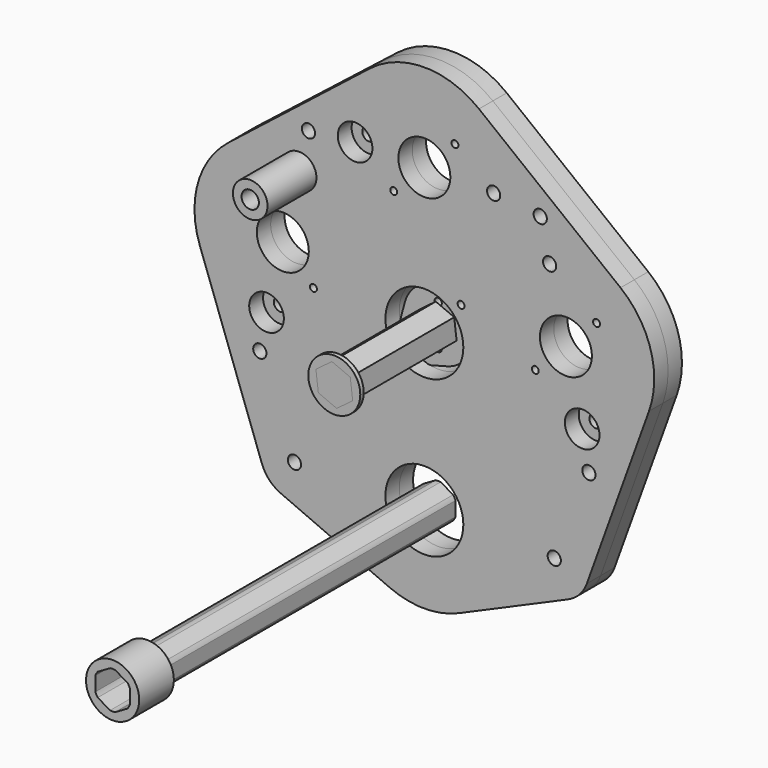
from build123d import *

# Parameters (mm, degrees)
F0_R      = 2.4257
F0_R_2    = 1.27
F0_R_3    = 14.2875
F0_R_4    = 9.525
F1_DEPTH  = 6.35
F2_R      = 6.35
F2_R_2    = 3.175
F3_DEPTH  = 28.7528
F5_DEPTH  = 47.625
F6_R      = 2.5527
F7_DEPTH  = 133.35
F8_R      = 2.4257
F8_R_2    = 6.35
F8_R_3    = 1.27
F8_R_4    = 14.2875
F8_R_5    = 9.525
F9_DEPTH  = 6.35
F10_R     = 9.7536
F11_DEPTH = 15.875
F12_R     = 9.525
F13_DEPTH = 1.5875
F14_R     = 1.3208
F14_R_2   = 1.27
F14_R_3   = 4.7625
F15_DEPTH = 3.175
F16_R     = 3.175
F16_R_2   = 1.27
F17_DEPTH = 6.35


with BuildPart() as f1:
    # F0 (on Front) → F1 (new body)
    with BuildSketch(Plane.XZ):
        with BuildLine():
            ThreePointArc((20.0287821123, 78.8394956856), (0, 85.7758), (-20.0287821123, 78.8394956856))
            Line((-20.0287821123, 78.8394956856), (-71.9241615496, 37.9964890253))
            ThreePointArc((-71.9241615496, 37.9964890253), (-83.0312055128, 21.4555741857), (-82.3532815297, 1.5430477664))
            Line((-82.3532815297, 1.5430477664), (-59.5692753303, -61.5163864993))
            ThreePointArc((-59.5692753303, -61.5163864993), (-56.8914611396, -65.8854242261), (-52.705, -68.8405422652))
            Line((-52.705, -68.8405422652), (-12.7, -86.300155663))
            ThreePointArc((-12.7, -86.300155663), (0, -88.9508), (12.7, -86.300155663))
            Line((12.7, -86.300155663), (52.705, -68.8405422652))
            ThreePointArc((52.705, -68.8405422652), (56.8914611396, -65.8854242261), (59.5692753303, -61.5163864993))
            Line((59.5692753303, -61.5163864993), (82.3532815297, 1.5430477664))
            ThreePointArc((82.3532815297, 1.5430477664), (83.0312055128, 21.4555741857), (71.9241615496, 37.9964890253))
            Line((71.9241615496, 37.9964890253), (20.0287821123, 78.8394956856))
        make_face()
        with Locations((-47.625, -57.2008)):
            Circle(F0_R, mode=Mode.SUBTRACT)
        with Locations((-60.325, -25.4508)):
            Circle(F0_R, mode=Mode.SUBTRACT)
        with Locations((-57.8648339281, -12.1407791805)):
            Circle(F0_R, mode=Mode.SUBTRACT)
        with Locations((-13.4703841816, -13.4703841816)):
            Circle(F0_R_2, mode=Mode.SUBTRACT)
        with Locations((0, -57.2008)):
            Circle(F0_R_3, mode=Mode.SUBTRACT)
        with Locations((47.625, -57.2008)):
            Circle(F0_R, mode=Mode.SUBTRACT)
        with Locations((60.325, -25.4508)):
            Circle(F0_R, mode=Mode.SUBTRACT)
        with Locations((57.8648339281, -12.1407791805)):
            Circle(F0_R, mode=Mode.SUBTRACT)
        with Locations((-51.8953794373, 12.5477933397)):
            Circle(F0_R_4, mode=Mode.SUBTRACT)
        with Locations((-63.1206995887, 23.773113491)):
            Circle(F0_R_2, mode=Mode.SUBTRACT)
        with Locations((-45.9259249465, 37.2363658598)):
            Circle(F0_R, mode=Mode.SUBTRACT)
        with Locations((-40.670059286, 1.3224731883)):
            Circle(F0_R_2, mode=Mode.SUBTRACT)
        with Locations((-42.4934886143, 51.4322950589)):
            Circle(F0_R, mode=Mode.SUBTRACT)
        with Locations((-25.4, 53.3908)):
            Circle(F0_R, mode=Mode.SUBTRACT)
        with Locations((-11.2253201513, 42.1654798487)):
            Circle(F0_R_2, mode=Mode.SUBTRACT)
        Circle(F0_R_3, mode=Mode.SUBTRACT)
        with Locations((13.4703841816, 13.4703841816)):
            Circle(F0_R_2, mode=Mode.SUBTRACT)
        with Locations((40.670059286, 1.3224731883)):
            Circle(F0_R_2, mode=Mode.SUBTRACT)
        with Locations((51.8953794373, 12.5477933397)):
            Circle(F0_R_4, mode=Mode.SUBTRACT)
        with Locations((63.1206995887, 23.773113491)):
            Circle(F0_R_2, mode=Mode.SUBTRACT)
        with Locations((45.9259249465, 37.2363658598)):
            Circle(F0_R, mode=Mode.SUBTRACT)
        with Locations((0, 53.3908)):
            Circle(F0_R_4, mode=Mode.SUBTRACT)
        with Locations((25.4, 53.3908)):
            Circle(F0_R, mode=Mode.SUBTRACT)
        with Locations((11.2253201513, 64.6161201513)):
            Circle(F0_R_2, mode=Mode.SUBTRACT)
        with Locations((42.4934886143, 51.4322950589)):
            Circle(F0_R, mode=Mode.SUBTRACT)
    extrude(amount=F1_DEPTH)


with BuildPart() as f3:
    # F2 (on face) → F3 (new body)
    with BuildSketch(Plane.XZ.offset(6.35)):
        with Locations((-45.9259249465, 37.2363658598)):
            Circle(F2_R)
        with Locations((-45.9259249465, 37.2363658598)):
            Circle(F2_R_2, mode=Mode.SUBTRACT)
    extrude(amount=F3_DEPTH)


with BuildPart() as f5:
    # F4 (on face) → F5 (new body)
    with BuildSketch(Plane.XZ.offset(6.35)):
        Polygon((0.8878003498, -7.2784025632), (6.7471816936, -2.8703436252), (5.8593813438, 4.408058938), (-0.8878003498, 7.2784025632), (-6.7471816936, 2.8703436252), (-5.8593813438, -4.408058938), align=None)
    extrude(amount=F5_DEPTH)


with BuildPart() as f7:
    # F6 (on face) → F7 (new body)
    with BuildSketch(Plane.XZ.offset(6.35)):
        with BuildLine():
            Line((0.8930394942, -64.0175518263), (5.4569605058, -61.3825708017))
            ThreePointArc((5.4569605058, -61.3825708017), (5.953924651, -60.6383), (6.35, -59.8357810246))
            Line((6.35, -59.8357810246), (6.35, -54.5658189754))
            ThreePointArc((6.35, -54.5658189754), (5.953924651, -53.7633), (5.4569605058, -53.0190291983))
            Line((5.4569605058, -53.0190291983), (0.8930394942, -50.3840481737))
            ThreePointArc((0.8930394942, -50.3840481737), (0, -50.3258), (-0.8930394942, -50.3840481737))
            Line((-0.8930394942, -50.3840481737), (-5.4569605058, -53.0190291983))
            ThreePointArc((-5.4569605058, -53.0190291983), (-5.953924651, -53.7633), (-6.35, -54.5658189754))
            Line((-6.35, -54.5658189754), (-6.35, -59.8357810246))
            ThreePointArc((-6.35, -59.8357810246), (-5.953924651, -60.6383), (-5.4569605058, -61.3825708017))
            Line((-5.4569605058, -61.3825708017), (-0.8930394942, -64.0175518263))
            ThreePointArc((-0.8930394942, -64.0175518263), (0, -64.0758), (0.8930394942, -64.0175518263))
        make_face()
        with Locations((0, -57.2008)):
            Circle(F6_R, mode=Mode.SUBTRACT)
    extrude(amount=F7_DEPTH)


with BuildPart() as f9:
    # F8 (on face) → F9 (new body)
    with BuildSketch(Plane.XZ.offset(6.35)):
        with BuildLine():
            Line((59.5692753303, -61.5163864993), (82.3532815297, 1.5430477664))
            ThreePointArc((82.3532815297, 1.5430477664), (83.0312055128, 21.4555741857), (71.9241615496, 37.9964890253))
            Line((71.9241615496, 37.9964890253), (20.0287821123, 78.8394956856))
            ThreePointArc((20.0287821123, 78.8394956856), (0, 85.7758), (-20.0287821123, 78.8394956856))
            Line((-20.0287821123, 78.8394956856), (-71.9241615496, 37.9964890253))
            ThreePointArc((-71.9241615496, 37.9964890253), (-83.0312055128, 21.4555741857), (-82.3532815297, 1.5430477664))
            Line((-82.3532815297, 1.5430477664), (-59.5692753303, -61.5163864993))
            ThreePointArc((-59.5692753303, -61.5163864993), (-56.8914611396, -65.8854242261), (-52.705, -68.8405422652))
            Line((-52.705, -68.8405422652), (-12.7, -86.300155663))
            ThreePointArc((-12.7, -86.300155663), (0, -88.9508), (12.7, -86.300155663))
            Line((12.7, -86.300155663), (52.705, -68.8405422652))
            ThreePointArc((52.705, -68.8405422652), (56.8914611396, -65.8854242261), (59.5692753303, -61.5163864993))
        make_face()
        with Locations((-47.625, -57.2008)):
            Circle(F8_R, mode=Mode.SUBTRACT)
        with Locations((-60.325, -25.4508)):
            Circle(F8_R, mode=Mode.SUBTRACT)
        with Locations((-57.8648339281, -12.1407791805)):
            Circle(F8_R_2, mode=Mode.SUBTRACT)
        with Locations((-13.4703841816, -13.4703841816)):
            Circle(F8_R_3, mode=Mode.SUBTRACT)
        with Locations((0, -57.2008)):
            Circle(F8_R_4, mode=Mode.SUBTRACT)
        with Locations((47.625, -57.2008)):
            Circle(F8_R, mode=Mode.SUBTRACT)
        with Locations((60.325, -25.4508)):
            Circle(F8_R, mode=Mode.SUBTRACT)
        with Locations((57.8648339281, -12.1407791805)):
            Circle(F8_R_2, mode=Mode.SUBTRACT)
        with Locations((-51.8953794373, 12.5477933397)):
            Circle(F8_R_5, mode=Mode.SUBTRACT)
        with Locations((-63.1206995887, 23.773113491)):
            Circle(F8_R_3, mode=Mode.SUBTRACT)
        with Locations((-45.9259249465, 37.2363658598)):
            Circle(F8_R, mode=Mode.SUBTRACT)
        with Locations((-40.670059286, 1.3224731883)):
            Circle(F8_R_3, mode=Mode.SUBTRACT)
        with Locations((-42.4934886143, 51.4322950589)):
            Circle(F8_R, mode=Mode.SUBTRACT)
        with Locations((-25.4, 53.3908)):
            Circle(F8_R_2, mode=Mode.SUBTRACT)
        with Locations((-11.2253201513, 42.1654798487)):
            Circle(F8_R_3, mode=Mode.SUBTRACT)
        Circle(F8_R_4, mode=Mode.SUBTRACT)
        with Locations((13.4703841816, 13.4703841816)):
            Circle(F8_R_3, mode=Mode.SUBTRACT)
        with Locations((40.670059286, 1.3224731883)):
            Circle(F8_R_3, mode=Mode.SUBTRACT)
        with Locations((51.8953794373, 12.5477933397)):
            Circle(F8_R_5, mode=Mode.SUBTRACT)
        with Locations((63.1206995887, 23.773113491)):
            Circle(F8_R_3, mode=Mode.SUBTRACT)
        with Locations((45.9259249465, 37.2363658598)):
            Circle(F8_R, mode=Mode.SUBTRACT)
        with Locations((0, 53.3908)):
            Circle(F8_R_5, mode=Mode.SUBTRACT)
        with Locations((25.4, 53.3908)):
            Circle(F8_R, mode=Mode.SUBTRACT)
        with Locations((11.2253201513, 64.6161201513)):
            Circle(F8_R_3, mode=Mode.SUBTRACT)
        with Locations((42.4934886143, 51.4322950589)):
            Circle(F8_R, mode=Mode.SUBTRACT)
    extrude(amount=F9_DEPTH)


with BuildPart() as f11:
    # F10 (on face) → F11 (new body)
    with BuildSketch(Plane.XZ.offset(139.7)):
        with Locations((0, -57.2008)):
            Circle(F10_R)
        with BuildLine():
            Line((-5.4569605058, -53.0190291983), (-0.8930394942, -50.3840481737))
            ThreePointArc((-0.8930394942, -50.3840481737), (0, -50.3258), (0.8930394942, -50.3840481737))
            Line((0.8930394942, -50.3840481737), (5.4569605058, -53.0190291983))
            ThreePointArc((5.4569605058, -53.0190291983), (5.953924651, -53.7633), (6.35, -54.5658189754))
            Line((6.35, -54.5658189754), (6.35, -59.8357810246))
            ThreePointArc((6.35, -59.8357810246), (5.953924651, -60.6383), (5.4569605058, -61.3825708017))
            Line((5.4569605058, -61.3825708017), (0.8930394942, -64.0175518263))
            ThreePointArc((0.8930394942, -64.0175518263), (0, -64.0758), (-0.8930394942, -64.0175518263))
            Line((-0.8930394942, -64.0175518263), (-5.4569605058, -61.3825708017))
            ThreePointArc((-5.4569605058, -61.3825708017), (-5.953924651, -60.6383), (-6.35, -59.8357810246))
            Line((-6.35, -59.8357810246), (-6.35, -54.5658189754))
            ThreePointArc((-6.35, -54.5658189754), (-5.953924651, -53.7633), (-5.4569605058, -53.0190291983))
        make_face(mode=Mode.SUBTRACT)
    extrude(amount=F11_DEPTH)


with BuildPart() as f13:
    # F12 (on face) → F13 (new body)
    with BuildSketch(Plane.XZ.offset(53.975)):
        Circle(F12_R)
        Polygon((5.8593813438, 4.408058938), (6.7471816936, -2.8703436252), (0.8878003498, -7.2784025632), (-5.8593813438, -4.408058938), (-6.7471816936, 2.8703436252), (-0.8878003498, 7.2784025632), align=None, mode=Mode.SUBTRACT)
    extrude(amount=-F13_DEPTH)


with BuildPart() as f15:
    # F14 (on face) → F15 (new body)
    with BuildSketch(Plane(origin=(0, -6.35, 0), x_dir=(-1, 0, 0), z_dir=(0, 1, 0))):
        with BuildLine():
            ThreePointArc((-12.6486337134, 16.5371986801), (-15.7154482119, 15.7154482119), (-16.5371986801, 12.6486337134))
            Line((-16.5371986801, 12.6486337134), (-12.2672579939, -3.2870018728))
            ThreePointArc((-12.2672579939, -3.2870018728), (-8.9802561211, -8.9802561211), (-3.2870018728, -12.2672579939))
            Line((-3.2870018728, -12.2672579939), (12.6486337134, -16.5371986801))
            ThreePointArc((12.6486337134, -16.5371986801), (15.7154482119, -15.7154482119), (16.5371986801, -12.6486337134))
            Line((16.5371986801, -12.6486337134), (12.2672579939, 3.2870018728))
            ThreePointArc((12.2672579939, 3.2870018728), (8.9802561211, 8.9802561211), (3.2870018728, 12.2672579939))
            Line((3.2870018728, 12.2672579939), (-12.6486337134, 16.5371986801))
        make_face()
        with Locations((0, -7.4422)):
            Circle(F14_R, mode=Mode.SUBTRACT)
        with Locations((13.4703841816, -13.4703841816)):
            Circle(F14_R_2, mode=Mode.SUBTRACT)
        Circle(F14_R_3, mode=Mode.SUBTRACT)
        with Locations((0, 7.4422)):
            Circle(F14_R, mode=Mode.SUBTRACT)
        with Locations((-13.4703841816, 13.4703841816)):
            Circle(F14_R_2, mode=Mode.SUBTRACT)
    extrude(amount=F15_DEPTH)

    # F16 (on face) → F17 (join)
    with BuildSketch(Plane(origin=(0, -3.175, 0), x_dir=(-1, 0, 0), z_dir=(0, 1, 0))):
        with Locations((-13.4703841816, 13.4703841816)):
            Circle(F16_R)
        with Locations((-13.4703841816, 13.4703841816)):
            Circle(F16_R_2, mode=Mode.SUBTRACT)
        with Locations((13.4703841816, -13.4703841816)):
            Circle(F16_R)
        with Locations((13.4703841816, -13.4703841816)):
            Circle(F16_R_2, mode=Mode.SUBTRACT)
    extrude(amount=F17_DEPTH)


solid = Compound([f1.part, f3.part, f5.part, f7.part, f9.part, f11.part, f13.part, f15.part])
